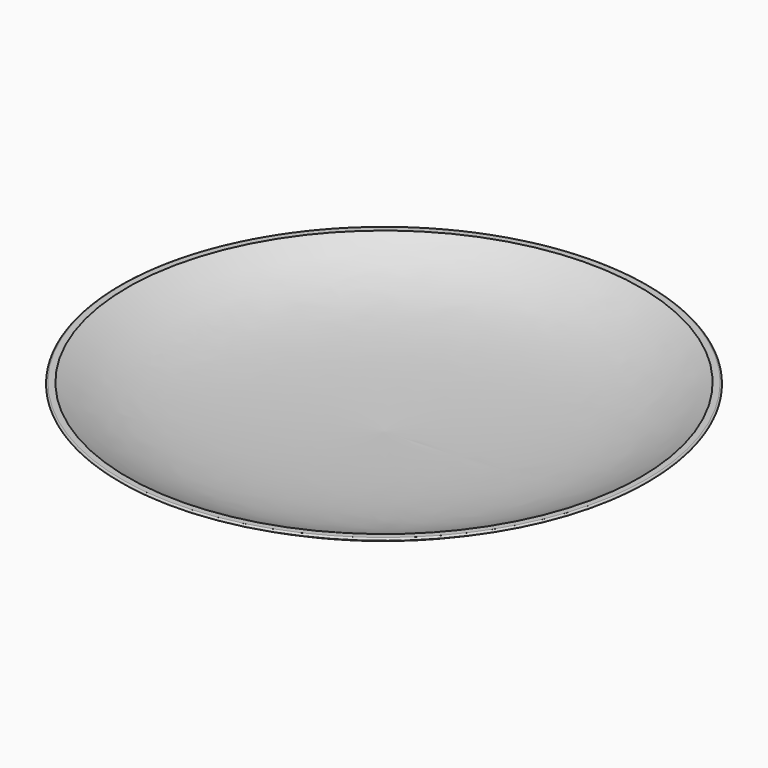
from build123d import *

# Parameters (mm, degrees)
F2_T = -1
F3_R = 0.25


with BuildPart() as f1:
    # F0 (on Front) → F1 (revolve)
    with BuildSketch(Plane.XZ):
        with BuildLine():
            Line((50, 9.1241644695), (0, 9.1241644695))
            Line((0, 9.1241644695), (0, 0))
            add(Edge.make_bspline(
                [(0, 0), (13.1994929815, 0.3230482128), (35.188760499, 0.8612199124), (45.7702564106, 6.7644607616), (50, 9.1241644695)],
                knots=[0, 0, 0, 0, 0.6002697894, 1, 1, 1, 1], degree=3))
        make_face()
    revolve(axis=Axis((0, 0, 4.5620822348), (0, 0, -1)))

    # F2
    f2_openings = [f1.faces().sort_by_distance(p)[0] for p in [
        (0, 0, 9.124164),
    ]]
    offset(amount=F2_T, openings=f2_openings)

    # F3
    f3_edges = [f1.edges().sort_by_distance(p)[0] for p in [
        (-50, 0, 9.124164),
    ]]
    fillet(f3_edges, radius=F3_R)


solid = f1.part
